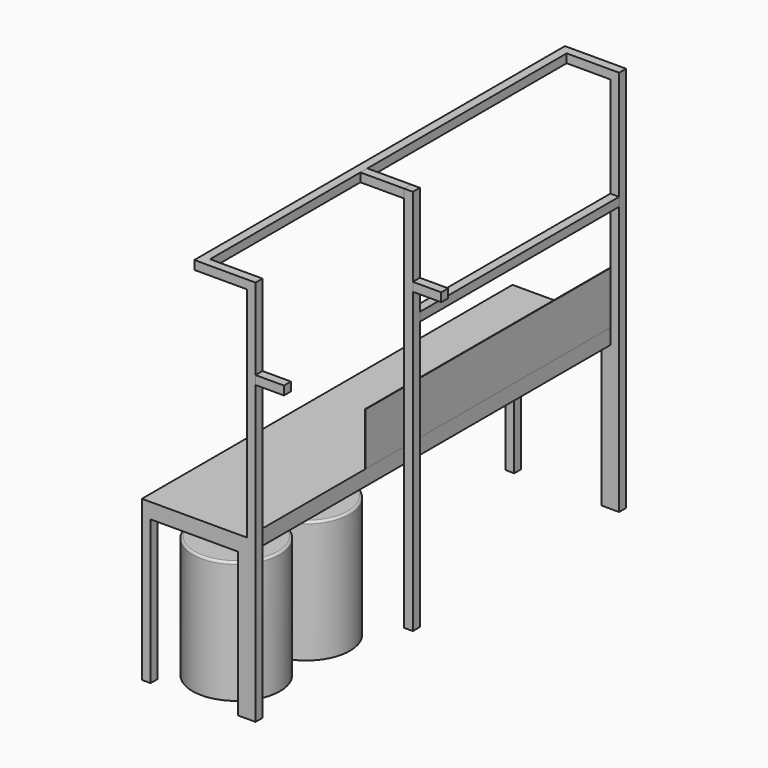
from build123d import *

# Parameters (mm, degrees)
F0_W      = 2692.4
F0_H      = 88.9
F1_DEPTH  = 609.6
F2_W      = 50.8
F2_H      = 50.8
F3_DEPTH  = 838.2
F5_DEPTH  = 711.2
F6_W      = 50.8
F6_H      = 50.8
F7_DEPTH  = 2247.9
F8_W      = 2692.4
F8_H      = 50.8
F9_DEPTH  = 304.8
F10_W     = 254
F10_H     = 2590.8
F11_DEPTH = 50.8
F12_W     = 3.175
F12_H     = 1778
F13_DEPTH = 304.8
F14_W     = 50.8
F14_H     = 50.8
F15_DEPTH = 2247.9
F16_T     = -25.4
F17_T     = -25.4
F18_R     = 12.69999
F19_R     = 12.69999
F20_W     = 50.8
F20_H     = 50.8
F21_DEPTH = 1447.8
F22_W     = 50.8
F22_H     = 50.8
F23_DEPTH = 165.1
F24_W     = 50.8
F24_H     = 50.8
F25_DEPTH = 254


# Not quite as in the source:
# - a fillet or chamfer is up to 0.001 mm smaller than in the source, because OpenCascade refuses the exact size


with BuildPart() as f1:
    # F0 (on Right) → F1 (new body)
    with BuildSketch(Plane.YZ):
        with Locations((5.8904625475, -73.3985408201)):
            Rectangle(F0_W, F0_H)
    extrude(amount=-F1_DEPTH)

    # F2 (on face) → F3 (join)
    with BuildSketch(Plane(origin=(0, 0, -117.8485408201), x_dir=(1, 0, 0), z_dir=(0, 0, -1))):
        with Locations((-584.2, 1314.9095374525)):
            Rectangle(F2_W, F2_H)
        with Locations((-25.4, 1314.9095374525)):
            Rectangle(F2_W, F2_H)
        with Locations((-25.4, -1326.6904625475)):
            Rectangle(F2_W, F2_H)
        with Locations((-584.2, -1326.6904625475)):
            Rectangle(F2_W, F2_H)
    extrude(amount=F3_DEPTH)

    # F6 (on face) → F7 (join)
    with BuildSketch(Plane(origin=(0, 0, -956.0485408201), x_dir=(1, 0, 0), z_dir=(0, 0, -1))):
        with Locations((25.4, 1314.9095374525)):
            Rectangle(F6_W, F6_H)
        with Locations((25.4, -1326.6904625475)):
            Rectangle(F6_W, F6_H)
    extrude(amount=-F7_DEPTH)

    # F8 (on face) → F9 (join)
    with BuildSketch(Plane(origin=(0, 0, 0), x_dir=(0, -1, 0), z_dir=(-1, 0, 0))):
        with Locations((-5.8904625475, 1266.4514591799)):
            Rectangle(F8_W, F8_H)
    extrude(amount=F9_DEPTH)

    # F10 (on face) → F11 (cut, through all)
    with BuildSketch(Plane.XY.offset(1291.8514591799)):
        with Locations((-127, 5.8904625475)):
            Rectangle(F10_W, F10_H)
    extrude(amount=-F11_DEPTH, mode=Mode.SUBTRACT)


with BuildPart() as f5:
    # F4 (on face) → F5 (new body)
    with BuildSketch(Plane(origin=(0, 0, -956.0485408201), x_dir=(1, 0, 0), z_dir=(0, 0, -1))):
        with BuildLine():
            ThreePointArc((-304.8, 781.5095374525), (-125.1948775786, 855.9044150311), (-50.8, 1035.5095374525))
            ThreePointArc((-50.8, 1035.5095374525), (-484.4051224214, 1215.1146598738), (-304.8, 781.5095374525))
        make_face()
    extrude(amount=-F5_DEPTH)

    # F17
    f17_openings = [f5.faces().sort_by_distance(p)[0] for p in [
        (-304.8, -1035.509537, -244.848541),
    ]]
    offset(amount=F17_T, openings=f17_openings)

    # F18 (radius 12.7 in the source; OpenCascade refuses exactly that, so slightly less here)
    f18_edges = [f5.edges().sort_by_distance(p)[0] for p in [
        (-304.8, -1289.509537, -244.848541),
        (-304.8, -1264.109537, -244.848541),
    ]]
    fillet(f18_edges, radius=F18_R)


with BuildPart() as f5b:
    # F4 (on face) → F5, piece 2 (new body)
    with BuildSketch(Plane(origin=(0, 0, -956.0485408201), x_dir=(1, 0, 0), z_dir=(0, 0, -1))):
        with BuildLine():
            ThreePointArc((-50.8, 527.5095374525), (-125.1948775786, 707.1146598738), (-304.8, 781.5095374525))
            ThreePointArc((-304.8, 781.5095374525), (-484.4051224214, 347.9044150311), (-50.8, 527.5095374525))
        make_face()
    extrude(amount=-F5_DEPTH)

    # F16
    f16_openings = [f5b.faces().sort_by_distance(p)[0] for p in [
        (-304.8, -527.509537, -244.848541),
    ]]
    offset(amount=F16_T, openings=f16_openings)

    # F19 (radius 12.7 in the source; OpenCascade refuses exactly that, so slightly less here)
    f19_edges = [f5b.edges().sort_by_distance(p)[0] for p in [
        (-558.8, -527.509537, -244.848541),
        (-533.4, -527.509537, -244.848541),
    ]]
    fillet(f19_edges, radius=F19_R)


with BuildPart() as f13:
    # F12 (on face) → F13 (new body)
    with BuildSketch(Plane.XY.offset(-28.9485408201)):
        with Locations((-1.5875, 412.2904625475)):
            Rectangle(F12_W, F12_H)
    extrude(amount=F13_DEPTH)


with BuildPart() as f15:
    # F14 (on face) → F15 (new body)
    with BuildSketch(Plane(origin=(0, 0, -956.0485408201), x_dir=(1, 0, 0), z_dir=(0, 0, -1))):
        with Locations((25.4, 171.9095374525)):
            Rectangle(F14_W, F14_H)
    extrude(amount=-F15_DEPTH)


with BuildPart() as f21:
    # F20 (on face) → F21 (new body, through all)
    with BuildSketch(Plane.XZ.offset(-1301.2904625475)):
        with Locations((25.4, 631.4514591799)):
            Rectangle(F20_W, F20_H)
    extrude(amount=F21_DEPTH)


with BuildPart() as f23:
    # F22 (on face) → F23 (new body)
    with BuildSketch(Plane.YZ.offset(50.8)):
        with Locations((-171.9095374525, 805.7018689156)):
            Rectangle(F22_W, F22_H)
    extrude(amount=F23_DEPTH)


with BuildPart() as f23b:
    # F22 (on face) → F23, piece 2 (new body)
    with BuildSketch(Plane.YZ.offset(50.8)):
        with Locations((-1314.9095374525, 793.3480314255)):
            Rectangle(F22_W, F22_H)
    extrude(amount=F23_DEPTH)


with BuildPart() as f25:
    # F24 (on face) → F25 (new body, through all)
    with BuildSketch(Plane(origin=(0, 0, 0), x_dir=(0, -1, 0), z_dir=(-1, 0, 0))):
        with Locations((171.9095374525, 1266.4514591799)):
            Rectangle(F24_W, F24_H)
    extrude(amount=F25_DEPTH)


solid = Compound([f1.part, f5.part, f5b.part, f13.part, f15.part, f21.part, f23.part, f23b.part, f25.part])
